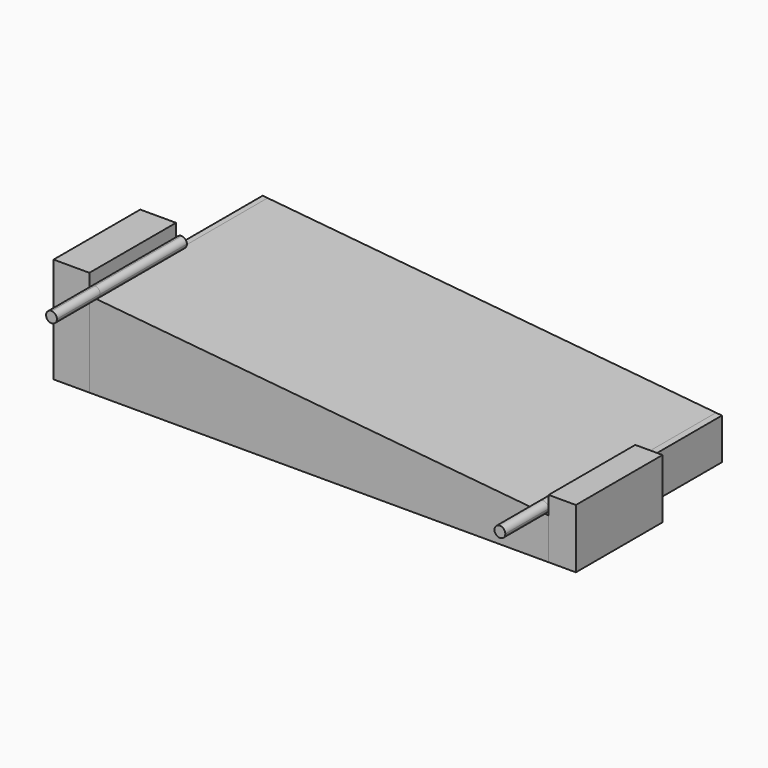
from build123d import *

# Parameters (mm, degrees)
F1_DEPTH      = 100
F2_DEPTH      = 25
F2_DEPTH_BACK = 50
F4_DEPTH      = 50


with BuildPart() as f1:
    # F0 (on Front) → F1 (new body)
    with BuildSketch(Plane.XZ):
        Polygon((0, 39.4), (0, 0), (212, 0), (212, 18.9867217821), (209.2603853098, 19.2505166731), (2.2603857104, 39.1823496114), align=None)
    extrude(amount=-F1_DEPTH)


with BuildPart() as f2:
    # F0 (on Front) → F2 (new body, two sides)
    with BuildSketch(Plane.XZ) as f2_sk:
        with BuildLine():
            ThreePointArc((2.5, 44.1708401161), (0.0028790316, 41.7907853914), (2.2603857104, 39.1823496114))
            ThreePointArc((2.2603857104, 39.1823496114), (4.1809170527, 39.8202948284), (5, 41.6708401161))
            ThreePointArc((5, 41.6708401161), (4.267766953, 43.4386070691), (2.5, 44.1708401161))
        make_face()
    extrude(amount=F2_DEPTH)
    extrude(f2_sk.sketch, amount=-F2_DEPTH_BACK)


with BuildPart() as f2b:
    # F0 (on Front) → F2, piece 2 (new body, two sides)
    with BuildSketch(Plane.XZ) as f2_2_sk:
        with BuildLine():
            ThreePointArc((212, 21.7390071392), (207.8190830963, 23.5895525623), (209.2603853098, 19.2505166731))
            ThreePointArc((209.2603853098, 19.2505166731), (211.1809169037, 19.8884617162), (212, 21.7390071392))
        make_face()
    extrude(amount=F2_DEPTH)
    extrude(f2_2_sk.sketch, amount=-F2_DEPTH_BACK)


with BuildPart() as f4:
    # F3 (on face) → F4 (new body)
    with BuildSketch(Plane.XZ):
        Polygon((212, 18.9867217821), (212, 0), (224.5859801769, 0), (224.5859801769, 27.3749008775), (212, 27.3749008775), align=None)
    extrude(amount=-F4_DEPTH)


with BuildPart() as f4b:
    # F3 (on face) → F4, piece 2 (new body)
    with BuildSketch(Plane.XZ):
        Polygon((-16.5345836431, 0), (0, 0), (0, 39.4), (0, 48.700671643), (-16.5345836431, 48.700671643), align=None)
    extrude(amount=-F4_DEPTH)


solid = Compound([f1.part, f2.part, f2b.part, f4.part, f4b.part])
